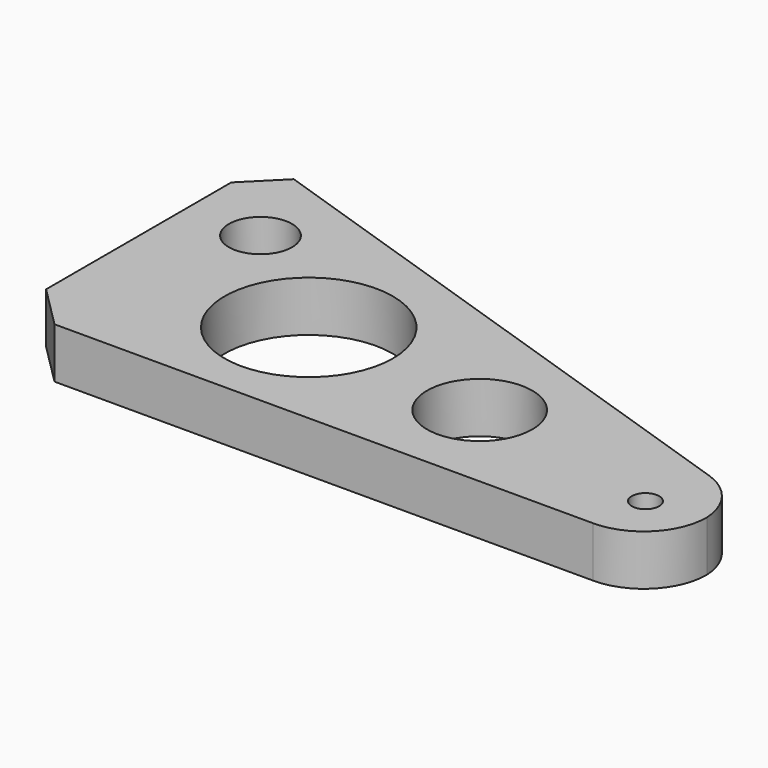
from build123d import *

# Parameters (mm, degrees)
F0_W        = 30.6
F0_H        = 15
F0_R        = 0.65
F1_DEPTH    = 2.4
F2_R        = 3
F3_SIZE     = 2
F4_T1_DEPTH = 158.1036606393
F5_T1_DEPTH = 13.1878115659
F6_R        = 1.5
F6_R_2      = 4
F6_R_3      = 2.5
F7_DEPTH    = 25


# Not quite as in the source:
# - a fillet or chamfer that OpenCascade refuses, or shapes differently, is made with other operations: its cross-section is extruded or revolved along the edge and cut away or added


with BuildPart() as f1:
    # F0 (on Top) → F1 (new body)
    with BuildSketch(Plane.XY):
        with Locations((15.3, 7.5)):
            Rectangle(F0_W, F0_H)
        with Locations((28, 2.6)):
            Circle(F0_R, mode=Mode.SUBTRACT)
    extrude(amount=F1_DEPTH)

    # F2
    f2_edges = [f1.edges().sort_by_distance(p)[0] for p in [
        (30.6, 0, 1.2),
    ]]
    fillet(f2_edges, radius=F2_R)

    # F3
    f3_edges = [f1.edges().sort_by_distance(p)[0] for p in [
        (0, 0, 1.2),
        (0, 15, 1.2),
    ]]
    chamfer(f3_edges, length=F3_SIZE)

    # F4: chamfer of 30 x 10 on 1 edges, made by hand

    # F4_s2 → F4_t1 (cut)
    with BuildSketch(Plane.XY.offset(-77.8518303197)):
        Polygon((30.6, 5), (0.6, 15), (30.6, 15), align=None)
    extrude(amount=F4_T1_DEPTH, mode=Mode.SUBTRACT)

    # F5: fillet of radius 3 on 1 edges, made by hand

    # F5_s2 → F5_t1 (cut)
    with BuildSketch(Plane.XY.offset(-5.3939057829)):
        with BuildLine():
            ThreePointArc((28.553156669, 5.6822811103), (29.9893960062, 4.6561608917), (30.6, 3))
            Line((30.6, 3), (30.6, 5))
            Line((30.6, 5), (28.553156669, 5.6822811103))
        make_face()
    extrude(amount=F5_T1_DEPTH, mode=Mode.SUBTRACT)

    # F6 (on face) → F7 (cut)
    with BuildSketch(Plane.XY.offset(2.4)):
        with Locations((3.5149192099, 10.3407332852)):
            Circle(F6_R)
        with Locations((9.5205735153, 5.6994225355)):
            Circle(F6_R_2)
        with Locations((18.6217441043, 4.476449427)):
            Circle(F6_R_3)
    extrude(amount=-F7_DEPTH, mode=Mode.SUBTRACT)


solid = f1.part
